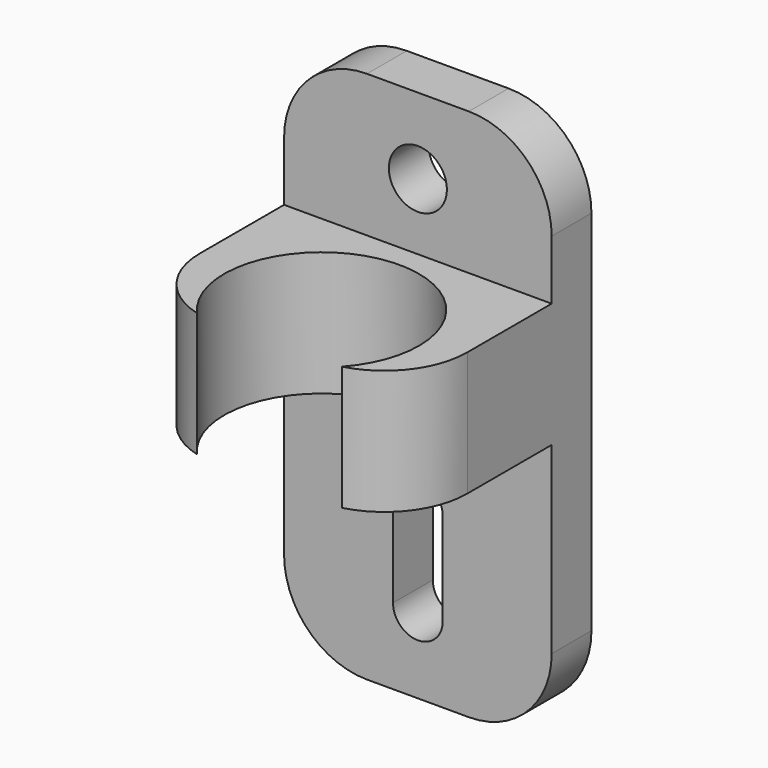
from build123d import *

# Parameters (mm, degrees)
F1_DEPTH    = 7.5
F2_W        = 16.1389429122
F2_H        = 16.083650291
F3_DEPTH    = 3
F4_D        = 3.5
F5_T1_DEPTH = 48.2954240112
F6_R        = 5


# Not quite as in the source:
# - a fillet or chamfer that OpenCascade refuses, or shapes differently, is made with other operations: its cross-section is extruded or revolved along the edge and cut away or added


with BuildPart() as f1:
    # F0 (on Top) → F1 (new body)
    with BuildSketch(Plane.XY):
        with BuildLine():
            ThreePointArc((-4.3675557451, -3.9293869513), (0, 5.875), (4.3675557451, -3.9293869513))
            Line((4.3675557451, -3.9293869513), (8.0694714561, -7.2599132545))
            Line((8.0694714561, -7.2599132545), (8.0694714561, 7.2599132545))
            Line((8.0694714561, 7.2599132545), (-8.0694714561, 7.2599132545))
            Line((-8.0694714561, 7.2599132545), (-8.0694714561, -7.2599132545))
            Line((-8.0694714561, -7.2599132545), (-4.3675557451, -3.9293869513))
        make_face()
    extrude(amount=F1_DEPTH)

    # F2 (on face) → F3 (join)
    with BuildSketch(Plane(origin=(0, 7.2599132545, 0), x_dir=(-1, 0, 0), z_dir=(0, 1, 0))):
        with Locations((0, -8.0418251455)):
            Rectangle(F2_W, F2_H)
        with BuildLine():
            Line((1.5, -5.9119383805), (1.5, -11.5))
            ThreePointArc((1.5, -11.5), (0, -13), (-1.5, -11.5))
            Line((-1.5, -11.5), (-1.5, -5.9119383805))
            ThreePointArc((-1.5, -5.9119383805), (0, -4.4119383805), (1.5, -5.9119383805))
        make_face(mode=Mode.SUBTRACT)
        with Locations((0, 8.0418251455)):
            Rectangle(F2_W, F2_H)
    extrude(amount=F3_DEPTH)

    # F4 (through all)
    with Locations(Plane(origin=(0, 7.2599132545, 0), x_dir=(-1, 0, 0), z_dir=(0, -1, 0))):
        with Locations((0, -11.5)):
            Hole(F4_D / 2)

    # F5: fillet of radius 5 on 2 edges, made by hand

    # F5_s2 → F5_t1 (cut)
    with BuildSketch(Plane.XY.offset(-20.3977120056)):
        with BuildLine():
            ThreePointArc((-8.0694714561, 0.8991715477), (-7.0374949846, -2.1429969679), (-4.3675557451, -3.9293869513))
            Line((-4.3675557451, -3.9293869513), (-8.0694714561, -7.2599132545))
            Line((-8.0694714561, -7.2599132545), (-8.0694714561, 0.8991715477))
        make_face()
        with BuildLine():
            ThreePointArc((8.0694714561, 0.8991715477), (7.0374949846, -2.1429969679), (4.3675557451, -3.9293869513))
            Line((4.3675557451, -3.9293869513), (8.0694714561, -7.2599132545))
            Line((8.0694714561, -7.2599132545), (8.0694714561, 0.8991715477))
        make_face()
    extrude(amount=F5_T1_DEPTH, mode=Mode.SUBTRACT)

    # F6
    f6_edges = [f1.edges().sort_by_distance(p)[0] for p in [
        (-8.069471, 8.759913, 16.08365),
        (8.069471, 8.759913, 16.08365),
        (8.069471, 8.759913, -16.08365),
        (-8.069471, 8.759913, -16.08365),
    ]]
    fillet(f6_edges, radius=F6_R)


solid = f1.part
